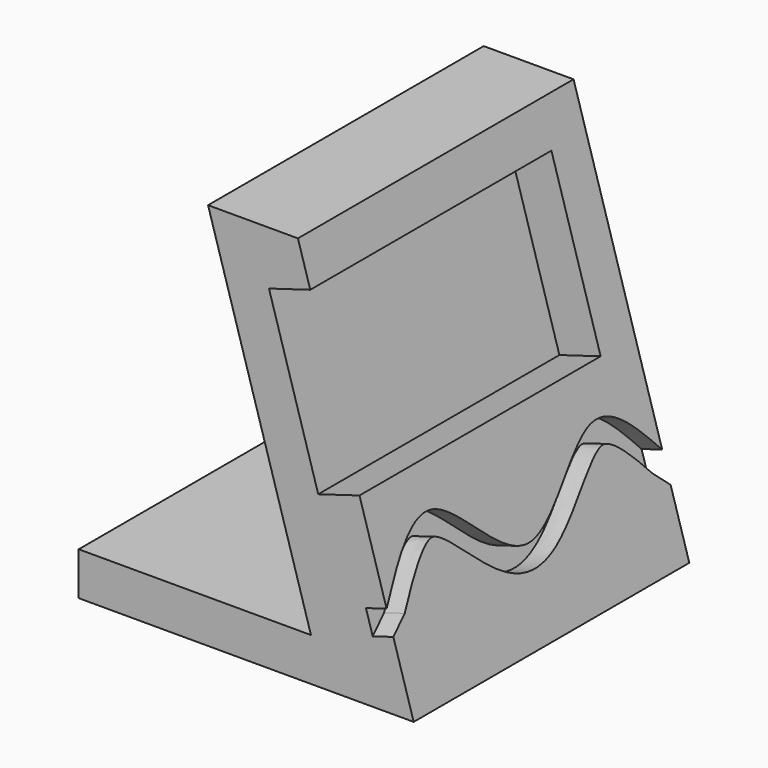
from build123d import *

# Parameters (mm, degrees)
F1_DEPTH = 40
F2_W     = 70
F2_H     = 40
F3_DEPTH = 10
F5_DEPTH = 5


# Not quite as in the source:
# - ends of sketch curves that miss each other by under 0.0002 mm in the source are joined
# - the dataset's text gives a spline's control points without its knots; the knots are read off the source's solid


with BuildPart() as f1:
    # F0 (on Front) → F1 (new body, symmetric)
    with BuildSketch(Plane.XZ):
        Polygon((-21.5449788049, -41.2119860854), (-21.5449788049, -51.2119860854), (35.3737750478, -51.2119860854), (32.3908216358, -41.2119860854), align=None)
        Polygon((32.3908216358, -41.2119860854), (35.3737750478, -51.2119860854), (56.2446170106, -51.2119860854), (29.3650766842, 38.8985071507), (8.4942347215, 38.8985071507), align=None)
    extrude(amount=F1_DEPTH, both=True)

    # F2 (on face) → F3 (cut)
    with BuildSketch(Plane(origin=(37.6208157973, 0, 11.2221140848), x_dir=(0, 1, 0), z_dir=(0.9582747086, 0, 0.2858488812))):
        with Locations((-5, -1.1185187112)):
            Rectangle(F2_W, F2_H)
    extrude(amount=-F3_DEPTH, mode=Mode.SUBTRACT)

    # F4 (on face) → F5 (cut)
    with BuildSketch(Plane(origin=(37.6208157973, 0, 11.2221140848), x_dir=(0, 1, 0), z_dir=(0.9582747086, 0, 0.2858488812))):
        with BuildLine():
            add(Edge.make_bspline(
                [(-40, -43.1355652991), (-34.2053294712, -36.0139301645), (-21.9622428705, -20.9672083092), (-0.3216553232, -58.7449573453), (23.1827234764, -22.5805966645), (34.6725355537, -36.6240552789), (40, -43.1355652991)],
                knots=[0, 0, 0, 0, 0.2381650355, 0.5031994727, 0.7696492224, 1, 1, 1, 1], degree=3))
            Line((-40, -43.1355652991), (-40, -48.6237816513))
            Line((-40, -48.6237816513), (-35.6619564775, -45.7264717672))
            add(Edge.make_bspline(
                [(-35.6619564775, -45.7264717672), (-35.0590566546, -44.9862360901), (-33.7171385936, -43.3447521589), (-31.6886989171, -40.9668012288), (-29.607364333, -38.760362672), (-27.6730019997, -37.0329619546), (-26.2737559313, -36.0960774678), (-25.3653436677, -35.6619003253), (-24.8066625548, -35.4756952703), (-24.3692440118, -35.398025809), (-24.0752323986, -35.3927631659), (-23.8452929972, -35.4170460505), (-23.6635270879, -35.4525110542), (-23.4652878515, -35.5086413181), (-23.1999390349, -35.6073921174), (-22.8784837278, -35.7543374211), (-22.3815687241, -36.0194215363), (-21.6506539435, -36.483137801), (-20.6451620675, -37.2377831197), (-19.1774270906, -38.4706699301), (-17.1622129865, -40.3563127024), (-14.5371565005, -42.9116720286), (-12.1784235459, -45.0862329058), (-10.1529440798, -46.7409148286), (-8.5454307599, -47.9101279594), (-6.8239101075, -48.9735311117), (-4.9550353669, -49.8858121237), (-3.2461184359, -50.4645187685), (-1.7828542729, -50.7696182934), (-0.6420654559, -50.9055898694), (0.5353388844, -50.9325928497), (1.6755135467, -50.850730431), (2.7789887973, -50.6755860925), (4.1927787493, -50.334925935), (5.8516627641, -49.7412199343), (7.6898739847, -48.8413633399), (9.4080407304, -47.8089144301), (11.5745061099, -46.3077948215), (14.1018131768, -44.277408327), (16.925590194, -41.8195528388), (19.1072870632, -39.9441867736), (20.7160812689, -38.6706168624), (21.8357201917, -37.8601616242), (22.842333558, -37.223537122), (23.6962630464, -36.7828118043), (24.2416400284, -36.5815699473), (24.5471222686, -36.5041182007), (24.7578339185, -36.4682045128), (24.9567697959, -36.4511243692), (25.2200453072, -36.4501488213), (25.5690606528, -36.48949836), (26.0751296049, -36.6241865888), (26.8930709535, -36.9623065426), (28.1729042903, -37.7450713905), (29.977280256, -39.2805705793), (31.9344365862, -41.3044708102), (33.9880373177, -43.6838767817), (35.4074362658, -45.4183375194), (36.1301742817, -46.3017063115)],
                knots=[0.006317439, 0.006317439, 0.006317439, 0.006317439, 0.03125, 0.0625, 0.09375, 0.125, 0.15625, 0.171875, 0.1875, 0.203125, 0.21875, 0.2265625, 0.234375, 0.2421875, 0.25, 0.2578125, 0.265625, 0.28125, 0.296875, 0.3125, 0.34375, 0.375, 0.40625, 0.421875, 0.4375, 0.453125, 0.46875, 0.484375, 0.4921875, 0.5, 0.5078125, 0.515625, 0.5234375, 0.53125, 0.546875, 0.5625, 0.578125, 0.59375, 0.625, 0.65625, 0.6875, 0.703125, 0.71875, 0.734375, 0.75, 0.765625, 0.7734375, 0.78125, 0.7890625, 0.796875, 0.8125, 0.828125, 0.84375, 0.875, 0.90625, 0.9375, 0.96875, 1, 1, 1, 1], degree=3))
            Line((36.1301742817, -46.3017063115), (40, -49.9784611166))
            Line((40, -49.9784611166), (40, -43.1355652991))
        make_face()
    extrude(amount=-F5_DEPTH, mode=Mode.SUBTRACT)


solid = f1.part
